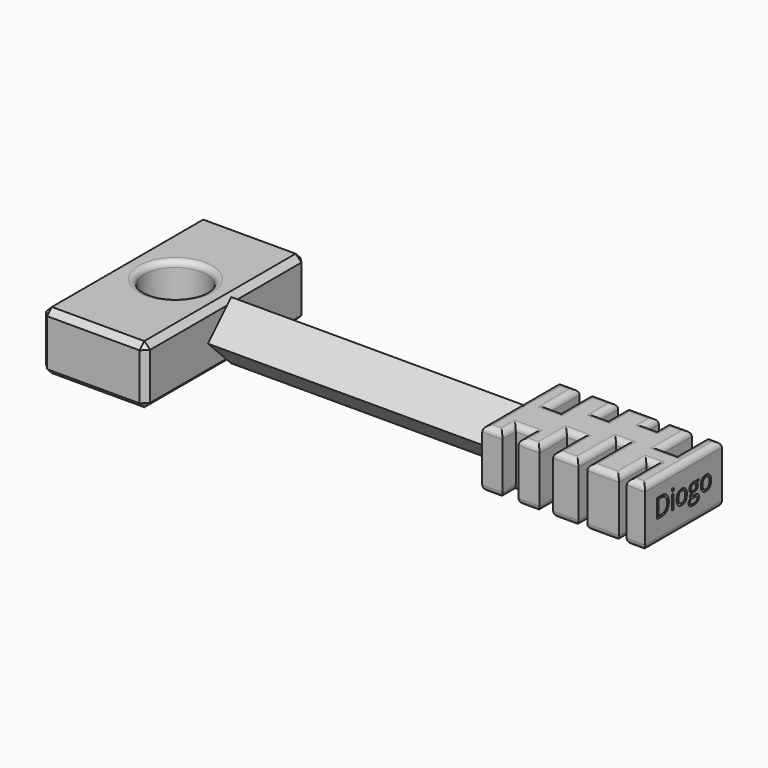
from build123d import *

# Parameters (mm, degrees)
F0_W          = 50
F0_H          = 10
F1_DEPTH      = 10
F2_W          = 17.8500991315
F2_H          = 34.4514474273
F3_DEPTH      = 10
F4_R          = 5.2772239771
F5_DEPTH      = 15
F6_SIZE       = 1
F7_W          = 27.9287863523
F7_H          = 16.4825590327
F8_DEPTH      = 10
F9_W          = 2.7563534677
F9_H          = 2.8503937647
F9_W_2        = 2.3526251316
F9_H_2        = 5.880090408
F9_W_3        = 1.5337318182
F9_H_3        = 8.088846691
F9_W_4        = 1.3261698186
F10_DEPTH     = 25
F11_W         = 2.0842254162
F11_H         = 6.5976213664
F11_W_2       = 1.7671138048
F11_H_2       = 4.3930821121
F11_W_3       = 1.7732828856
F11_H_3       = 2.6905909181
F11_W_4       = 2.7279779315
F12_DEPTH     = 25
F13_R         = 1
F14_SIZE      = 4.99999
F15_R         = 1
F16_TEXT_SIZE = 4.5007068871
F17_DEPTH     = 1


# Not quite as in the source:
# - a fillet or chamfer is up to 0.001 mm smaller than in the source, because OpenCascade refuses the exact size
# - Text() gives the source's letters only with a copy of the font that has no kerning and outlines rounded to 1/6400 em; it was checked with that copy


with BuildPart() as f1:
    # F0 (on Top) → F1 (new body)
    with BuildSketch(Plane.XY):
        with Locations((4.9076052383, 18.2365099943)):
            Rectangle(F0_W, F0_H)
    extrude(amount=F1_DEPTH)

    # F7 (on Top) → F8 (join)
    with BuildSketch(Plane.XY):
        with Locations((43.3811796829, 18.428416457)):
            Rectangle(F7_W, F7_H)
    extrude(amount=F8_DEPTH)

    # F9 (on face) → F10 (cut)
    with BuildSketch(Plane.XY.offset(10)):
        with Locations((34.2649836093, 11.612333823)):
            Rectangle(F9_W, F9_H)
        with Locations((40.4178388417, 13.1271821447)):
            Rectangle(F9_W_2, F9_H_2)
        with Locations((46.6744974256, 14.2315602861)):
            Rectangle(F9_W_3, F9_H_3)
        with Locations((53.5366740078, 13.1271821447)):
            Rectangle(F9_W_4, F9_H_2)
    extrude(amount=-F10_DEPTH, mode=Mode.SUBTRACT)

    # F11 (on face) → F12 (cut)
    with BuildSketch(Plane(origin=(0, 0, 0), x_dir=(1, 0, 0), z_dir=(0, 0, -1))):
        with Locations((33.9606739581, -23.3708852902)):
            Rectangle(F11_W, F11_H)
        with Locations((40.4414348304, -24.4731549174)):
            Rectangle(F11_W_2, F11_H_2)
        with Locations((47.4065579474, -25.3244005144)):
            Rectangle(F11_W_3, F11_H_3)
        with Locations((53.5511411726, -23.3708852902)):
            Rectangle(F11_W_4, F11_H)
    extrude(amount=-F12_DEPTH, mode=Mode.SUBTRACT)

    # F14 (size 5 in the source; OpenCascade refuses exactly that, so slightly less here)
    f14_edges = [f1.edges().sort_by_distance(p)[0] for p in [
        (4.662196, 23.23651, 0),
        (4.662196, 13.23651, 0),
        (4.662196, 13.23651, 10),
        (4.662196, 23.23651, 10),
    ]]
    chamfer(f14_edges, length=F14_SIZE)

    # F15
    f15_edges = [f1.edges().sort_by_distance(p)[0] for p in [
        (55.772666, 10.187137, 10),
        (50.157476, 10.187137, 10),
        (43.750891, 10.187137, 10),
        (37.442343, 10.187137, 10),
        (34.264984, 13.037531, 10),
        (31.151797, 10.187137, 10),
        (32.886807, 11.612334, 10),
        (39.241526, 13.127182, 10),
        (40.417839, 16.067227, 10),
        (41.594151, 13.127182, 10),
        (35.64316, 11.612334, 10),
        (47.441363, 14.23156, 10),
        (29.416787, 20.736515, 10),
        (29.416787, 15.736505, 10),
        (29.416787, 24.953103, 10),
        (29.416787, 11.711823, 10),
        (31.167674, 26.669696, 10),
        (32.918561, 23.370885, 10),
        (33.960674, 20.072075, 10),
        (35.002787, 23.370885, 10),
        (37.280332, 26.669696, 10),
        (39.557878, 24.473155, 10),
        (40.441435, 22.276614, 10),
        (41.324992, 24.473155, 10),
        (43.922454, 26.669696, 10),
        (46.519917, 25.324401, 10),
        (45.907632, 14.23156, 10),
        (47.406558, 23.979105, 10),
        (46.674497, 18.275984, 10),
        (48.293199, 25.324401, 10),
        (50.240176, 26.669696, 10),
        (52.187152, 23.370885, 10),
        (52.873589, 13.127182, 10),
        (53.551141, 20.072075, 10),
        (53.536674, 16.067227, 10),
        (54.91513, 23.370885, 10),
        (54.199759, 13.127182, 10),
        (56.130351, 26.669696, 10),
        (57.345573, 18.428416, 10),
        (29.416787, 20.736515, 0),
        (29.416787, 15.736505, 0),
        (29.416787, 24.953103, 0),
        (29.416787, 11.711823, 0),
        (31.167674, 26.669696, 0),
        (31.151797, 10.187137, 0),
        (32.918561, 23.370885, 0),
        (32.886807, 11.612334, 0),
        (33.960674, 20.072075, 0),
        (34.264984, 13.037531, 0),
        (35.002787, 23.370885, 0),
        (35.64316, 11.612334, 0),
        (37.280332, 26.669696, 0),
        (37.442343, 10.187137, 0),
        (39.557878, 24.473155, 0),
        (39.241526, 13.127182, 0),
        (40.441435, 22.276614, 0),
        (40.417839, 16.067227, 0),
        (41.324992, 24.473155, 0),
        (41.594151, 13.127182, 0),
        (43.922454, 26.669696, 0),
        (43.750891, 10.187137, 0),
        (46.519917, 25.324401, 0),
        (45.907632, 14.23156, 0),
        (47.406558, 23.979105, 0),
        (46.674497, 18.275984, 0),
        (48.293199, 25.324401, 0),
        (47.441363, 14.23156, 0),
        (50.240176, 26.669696, 0),
        (50.157476, 10.187137, 0),
        (52.187152, 23.370885, 0),
        (52.873589, 13.127182, 0),
        (53.551141, 20.072075, 0),
        (53.536674, 16.067227, 0),
        (54.91513, 23.370885, 0),
        (54.199759, 13.127182, 0),
        (56.130351, 26.669696, 0),
        (55.772666, 10.187137, 0),
        (57.345573, 18.428416, 0),
    ]]
    fillet(f15_edges, radius=F15_R)

    # F16 (on face) → F17 (cut)
    with BuildSketch(Plane.YZ.offset(57.345572859)):
        with Locations((12.285457924, 3.8668471389)):
            Text('Diogo', F16_TEXT_SIZE, font='Open Sans', text_align=(TextAlign.LEFT, TextAlign.BOTTOM))
    extrude(amount=-F17_DEPTH, mode=Mode.SUBTRACT)


with BuildPart() as f3:
    # F2 (on Top) → F3 (new body)
    with BuildSketch(Plane.XY):
        with Locations((-29.1290367022, 17.2257237136)):
            Rectangle(F2_W, F2_H)
    extrude(amount=F3_DEPTH)

    # F4 (on face) → F5 (cut)
    with BuildSketch(Plane.XY.offset(10)):
        with Locations((-29.1691944003, 17.6523067057)):
            Circle(F4_R)
    extrude(amount=-F5_DEPTH, mode=Mode.SUBTRACT)

    # F6
    f6_edges = [f3.edges().sort_by_distance(p)[0] for p in [
        (-20.203987, 17.225724, 10),
        (-29.129037, 0, 10),
        (-38.054086, 17.225724, 10),
        (-29.129037, 34.451447, 10),
        (-38.054086, 34.451447, 5),
        (-38.054086, 0, 5),
        (-20.203987, 0, 5),
        (-20.203987, 34.451447, 5),
        (-38.054086, 17.225724, 0),
        (-29.129037, 34.451447, 0),
        (-29.129037, 0, 0),
        (-20.203987, 17.225724, 0),
    ]]
    chamfer(f6_edges, length=F6_SIZE)

    # F13
    f13_edges = [f3.edges().sort_by_distance(p)[0] for p in [
        (-34.446418, 17.652307, 0),
        (-34.446418, 17.652307, 10),
        (-23.89197, 17.652307, 5),
    ]]
    fillet(f13_edges, radius=F13_R)


solid = Compound([f1.part, f3.part])
